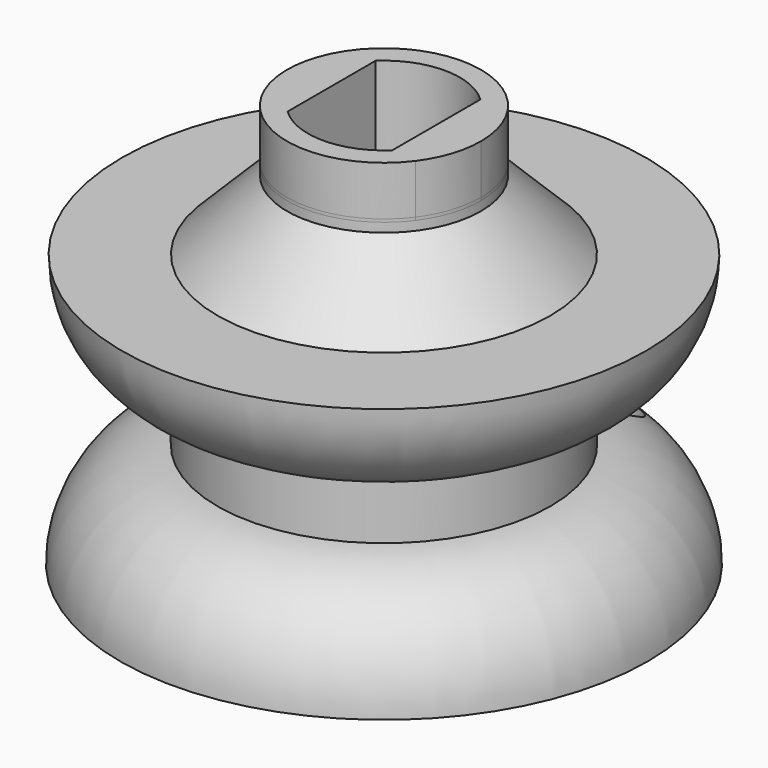
from build123d import *

# Parameters (mm, degrees)
F1_DEPTH    = 6.35
F2_R        = 12.6960047963
F2_R_2      = 8.0729751922
F3_DEPTH    = 5.08
F4_DEPTH    = 8.128
F5_R        = 12.7953112481
F5_R_2      = 1.3354653725
F5_R_3      = 8.0729751922
F6_DEPTH    = 5.08
F0_R        = 8.0645
F8_DEPTH    = 3.81
F9_S6_R     = 4.699
F9_T7_DEPTH = 39


# Not quite as in the source:
# - a fillet or chamfer that OpenCascade refuses, or shapes differently, is made with other operations: its cross-section is extruded or revolved along the edge and cut away or added


with BuildPart() as f1:
    # F0 (on Top) → F1 (new body)
    with BuildSketch(Plane.XY):
        with BuildLine():
            Line((-2.54, -2.8050532779), (-3.7699173874, -2.8050532779))
            ThreePointArc((-3.7699173874, -2.8050532779), (-0.0014195763, -4.6989997856), (3.7682218762, -2.8073305634))
            Line((3.7682218762, -2.8073305634), (2.54, -2.8073305634))
            Line((2.54, -2.8073305634), (2.54, -2.667))
            ThreePointArc((2.54, -2.667), (0, -3.683), (-2.54, -2.667))
            Line((-2.54, -2.667), (-2.54, -2.8050532779))
        make_face()
        with BuildLine():
            Line((2.54, 0), (2.54, -2.667))
            ThreePointArc((2.54, -2.667), (3.3852111456, -1.4508047767), (3.683, 0))
            ThreePointArc((3.683, 0), (3.3852111456, 1.4508047767), (2.54, 2.667))
            Line((2.54, 2.667), (2.54, 0))
        make_face()
        with BuildLine():
            Line((2.54, -2.8073305634), (3.7682218762, -2.8073305634))
            Line((3.7682218762, -2.8073305634), (3.7682218762, 2.667))
            Line((3.7682218762, 2.667), (2.54, 2.667))
            ThreePointArc((2.54, 2.667), (3.3852111456, 1.4508047767), (3.683, 0))
            ThreePointArc((3.683, 0), (3.3852111456, -1.4508047767), (2.54, -2.667))
            Line((2.54, -2.667), (2.54, -2.8073305634))
        make_face()
        with BuildLine():
            ThreePointArc((3.7682218762, -2.8073305634), (4.460239657, -1.4788046531), (4.699, 0))
            ThreePointArc((4.699, 0), (-1.4774571392, 4.460686203), (-3.7699173874, -2.8050532779))
            Line((-3.7699173874, -2.8050532779), (-3.7699173874, 2.667))
            Line((-3.7699173874, 2.667), (-2.54, 2.667))
            ThreePointArc((-2.54, 2.667), (0, 3.683), (2.54, 2.667))
            Line((2.54, 2.667), (3.7682218762, 2.667))
            Line((3.7682218762, 2.667), (3.7682218762, -2.8073305634))
        make_face()
        with BuildLine():
            Line((-3.7699173874, 2.667), (-3.7699173874, -2.8050532779))
            Line((-3.7699173874, -2.8050532779), (-2.54, -2.8050532779))
            Line((-2.54, -2.8050532779), (-2.54, -2.667))
            ThreePointArc((-2.54, -2.667), (-3.683, 0), (-2.54, 2.667))
            Line((-2.54, 2.667), (-3.7699173874, 2.667))
        make_face()
        with BuildLine():
            ThreePointArc((-2.54, 2.667), (-3.683, 0), (-2.54, -2.667))
            Line((-2.54, -2.667), (-2.54, 0))
            Line((-2.54, 0), (-2.54, 2.667))
        make_face()
    extrude(amount=F1_DEPTH)



with BuildPart() as f3:
    # F2 (on Top) → F3 (new body)
    with BuildSketch(Plane.XY):
        Circle(F2_R)
        Circle(F2_R_2, mode=Mode.SUBTRACT)
    extrude(amount=-F3_DEPTH)


with BuildPart() as f1_1:
    add(f1.part)

    add(f3.part)  # F4 merges F3
    # F2 (on Top) → F4 (join)
    with BuildSketch(Plane.XY):
        Circle(F2_R_2)
    extrude(amount=-F4_DEPTH)

    # F5 (on face) → F6 (join)
    with BuildSketch(Plane(origin=(0, 0, -8.128), x_dir=(1, 0, 0), z_dir=(0, 0, -1))):
        Circle(F5_R)
        with Locations((3.9191520773, -8.7972320383)):
            Circle(F5_R_2, mode=Mode.SUBTRACT)
        Circle(F5_R_3, mode=Mode.SUBTRACT)
        Circle(F5_R_3)
    extrude(amount=F6_DEPTH)

    # F7: fillet of radius 5.08 on 2 edges, made by hand

    # F7_s1 → F7_t2 (revolve, cut)
    with BuildSketch(Plane.XZ):
        with BuildLine():
            ThreePointArc((12.7953112481, -13.1953934624), (11.4317162877, -9.7320520727), (8.0729751922, -8.128))
            Line((8.0729751922, -8.128), (12.7953112481, -8.128))
            Line((12.7953112481, -8.128), (12.7953112481, -13.1953934624))
        make_face()
    revolve(axis=Axis((0, 0, -8.128), (0, 0, -1)), mode=Mode.SUBTRACT)

    # F7_s3 → F7_t4 (revolve, cut)
    with BuildSketch(Plane.XZ):
        with BuildLine():
            ThreePointArc((8.0729751922, -5.08), (11.366192099, -3.4473275256), (12.6960047963, -0.0205950886))
            Line((12.6960047963, -0.0205950886), (12.6960047963, -5.08))
            Line((12.6960047963, -5.08), (8.0729751922, -5.08))
        make_face()
    revolve(axis=Axis((0, 0, -5.08), (0, 0, 1)), mode=Mode.SUBTRACT)

    # F0 (on Top) → F8 (join)
    with BuildSketch(Plane.XY):
        Circle(F0_R)
        with BuildLine():
            ThreePointArc((-3.7699173874, -2.8050532779), (-1.4774571392, 4.460686203), (4.699, 0))
            ThreePointArc((4.699, 0), (4.460239657, -1.4788046531), (3.7682218762, -2.8073305634))
            ThreePointArc((3.7682218762, -2.8073305634), (-0.0014195763, -4.6989997856), (-3.7699173874, -2.8050532779))
        make_face(mode=Mode.SUBTRACT)
    extrude(amount=F8_DEPTH)

    # F9: chamfer of 3.81 on 1 edges, made by hand


with BuildPart() as f9_tool2:
    # F9_s3 → F9_t4 (revolve)
    with BuildSketch(Plane.XZ):
        with BuildLine():
            Line((8.1722630735, -0.1077630735), (4.1467369265, 3.9177630735))
            Line((4.1467369265, 3.9177630735), (4.1467369265, 3.9939630735))
            ThreePointArc((4.1467369265, 3.9939630735), (6.1056184633, 3.8862), (8.0645, 3.8862))
            Line((8.0645, 3.8862), (8.1407, 3.81))
            ThreePointArc((8.1407, 3.81), (8.1407, 1.8511184633), (8.2484630735, -0.1077630735))
            Line((8.2484630735, -0.1077630735), (8.1722630735, -0.1077630735))
        make_face()
    revolve(axis=Axis((0, 0, 3.81), (0, 0, 1)))

    split(bisect_by=Plane.XY, keep=Keep.TOP)

    # F9_s6 → F9_t7 (cut, symmetric)
    with BuildSketch(Plane.XY.offset(2.8)):
        Circle(F9_S6_R)
    extrude(amount=F9_T7_DEPTH, both=True, mode=Mode.SUBTRACT)


with BuildPart() as f1_2:
    add(f1_1.part)

    # F9_t1: cut F9_tool2
    add(f9_tool2.part, mode=Mode.SUBTRACT)


solid = f1_2.part
